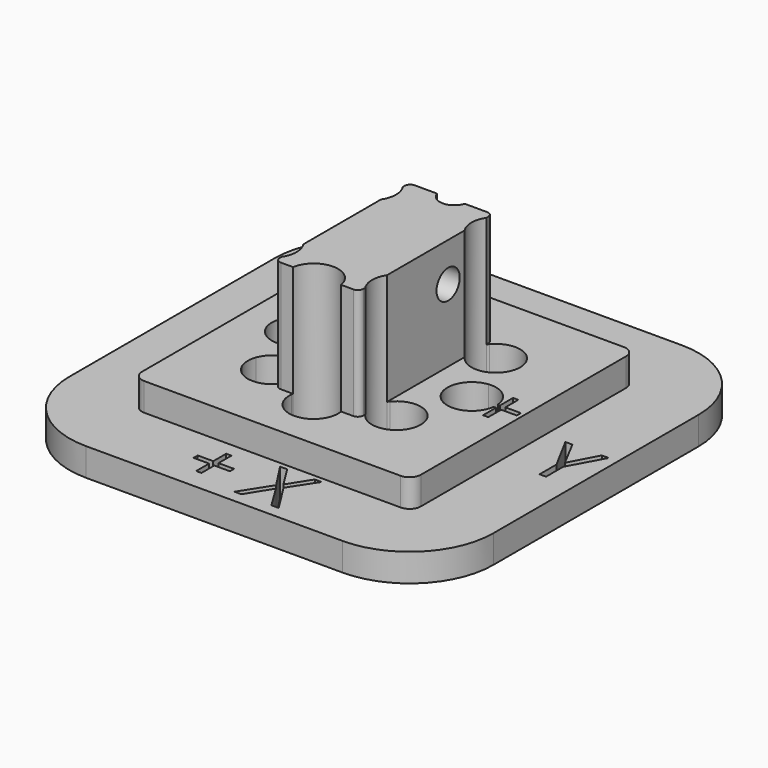
from build123d import *
from build123d import SkipClean  # not in build123d's __all__

# Parameters (mm, degrees)
F0_R      = 2.575
F1_DEPTH  = 10
F2_DEPTH  = 10
F4_START  = 5
F4_DEPTH  = 5
F7_DEPTH  = 30
F8_R      = 2.6
F9_DEPTH  = 12.5
F11_START = 5
F11_DEPTH = 5


# Not quite as in the source:
# - after a boolean that leaves OpenCascade's solid faulty, fix() repairs it


with BuildPart() as f1:
    # F0 (on Top) → F1 (new body)
    with BuildSketch(Plane.XY):
        with BuildLine():
            Line((23, 38), (-23, 38))
            ThreePointArc((-23, 38), (-33.6066017178, 33.6066017178), (-38, 23))
            Line((-38, 23), (-38, -23))
            ThreePointArc((-38, -23), (-33.6066017178, -33.6066017178), (-23, -38))
            Line((-23, -38), (23, -38))
            ThreePointArc((23, -38), (33.6066017178, -33.6066017178), (38, -23))
            Line((38, -23), (38, 23))
            ThreePointArc((38, 23), (33.6066017178, 33.6066017178), (23, 38))
        make_face()
        Polygon((-5.3266059028, -27.5300209804), (-5.3266059028, -30.4314966748), (-2.5336371528, -30.4314966748), (-2.5336371528, -31.3668265359), (-5.3266059028, -31.3668265359), (-5.3266059028, -34.2574515359), (-6.2706163194, -34.2574515359), (-6.2706163194, -31.3668265359), (-9.0505642361, -31.3668265359), (-9.0505642361, -30.4314966748), (-6.2706163194, -30.4314966748), (-6.2706163194, -27.5300209804), align=None, mode=Mode.SUBTRACT)
        Polygon((6.4463975694, -30.5747258415), (9.755859375, -35.7960800081), (8.447265625, -35.7960800081), (5.7823350694, -31.4362709804), (3.0696614583, -35.7960800081), (1.8478732639, -35.7960800081), (5.1443142361, -30.6137883415), (2.0713975694, -25.8807154248), (3.3474392361, -25.8807154248), (5.8083767361, -29.8086668137), (8.291015625, -25.8807154248), (9.5171440972, -25.8807154248), align=None, mode=Mode.SUBTRACT)
        Polygon((29.8459162505, 4.9153645833), (32.4717843061, -0.0434027778), (35.1150134727, 4.9153645833), (36.3628433338, 4.9153645833), (33.0533815283, -1.1545138889), (33.0533815283, -5), (31.888016945, -5), (31.888016945, -1.2087673611), (28.5850655561, 4.9153645833), align=None, mode=Mode.SUBTRACT)
        with BuildLine():
            ThreePointArc((-25, 23), (-24.4142135624, 24.4142135624), (-23, 25))
            Line((-23, 25), (23, 25))
            ThreePointArc((23, 25), (24.4142135624, 24.4142135624), (25, 23))
            Line((25, 23), (25, -23))
            ThreePointArc((25, -23), (24.4142135624, -24.4142135624), (23, -25))
            Line((23, -25), (-23, -25))
            ThreePointArc((-23, -25), (-24.4142135624, -24.4142135624), (-25, -23))
            Line((-25, -23), (-25, 23))
        make_face(mode=Mode.SUBTRACT)
        with BuildLine():
            Line((23, 25), (-23, 25))
            ThreePointArc((-23, 25), (-24.4142135624, 24.4142135624), (-25, 23))
            Line((-25, 23), (-25, -23))
            ThreePointArc((-25, -23), (-24.4142135624, -24.4142135624), (-23, -25))
            Line((-23, -25), (23, -25))
            ThreePointArc((23, -25), (24.4142135624, -24.4142135624), (25, -23))
            Line((25, -23), (25, 23))
            ThreePointArc((25, 23), (24.4142135624, 24.4142135624), (23, 25))
        make_face()
        with BuildLine():
            ThreePointArc((-15.25, 9.6458600373), (-15.5119318037, 11.1369318037), (-15.25, 12.6280035701))
            Line((-15.25, 12.6280035701), (-15.25, 14))
            ThreePointArc((-15.25, 14), (-12.6871843354, 20.1871843354), (-6.5, 22.75))
            Line((-6.5, 22.75), (6.5, 22.75))
            ThreePointArc((6.5, 22.75), (12.6871843354, 20.1871843354), (15.25, 14))
            Line((15.25, 14), (15.25, 12.6280035701))
            ThreePointArc((15.25, 12.6280035701), (15.4459513185, 11.893883467), (15.5119318037, 11.1369318037))
            ThreePointArc((15.5119318037, 11.1369318037), (15.4459513185, 10.3799801404), (15.25, 9.6458600373))
            Line((15.25, 9.6458600373), (15.25, 4.3463346627))
            ThreePointArc((15.25, 4.3463346627), (18.5227362424, 3.384162929), (20.1097825626, 0.3645833333))
            Line((20.1097825626, 0.3645833333), (20.520829445, 0.3645833333))
            Line((20.520829445, 0.3645833333), (20.520829445, 3.2660590278))
            Line((20.520829445, 3.2660590278), (21.4648398616, 3.2660590278))
            Line((21.4648398616, 3.2660590278), (21.4648398616, 0.3645833333))
            Line((21.4648398616, 0.3645833333), (24.2578086116, 0.3645833333))
            Line((24.2578086116, 0.3645833333), (24.2578086116, -0.5707465278))
            Line((24.2578086116, -0.5707465278), (21.4648398616, -0.5707465278))
            Line((21.4648398616, -0.5707465278), (21.4648398616, -3.4613715278))
            Line((21.4648398616, -3.4613715278), (20.520829445, -3.4613715278))
            Line((20.520829445, -3.4613715278), (20.520829445, -0.5707465278))
            Line((20.520829445, -0.5707465278), (20.0876114857, -0.5707465278))
            ThreePointArc((20.0876114857, -0.5707465278), (18.4417618617, -3.4489191176), (15.25, -4.3463346627))
            Line((15.25, -4.3463346627), (15.25, -9.6458600373))
            ThreePointArc((15.25, -9.6458600373), (15.4459513185, -10.3799801404), (15.5119318037, -11.1369318037))
            ThreePointArc((15.5119318037, -11.1369318037), (15.4459513185, -11.893883467), (15.25, -12.6280035701))
            Line((15.25, -12.6280035701), (15.25, -14))
            ThreePointArc((15.25, -14), (12.6871843354, -20.1871843354), (6.5, -22.75))
            Line((6.5, -22.75), (-6.5, -22.75))
            ThreePointArc((-6.5, -22.75), (-12.6871843354, -20.1871843354), (-15.25, -14))
            Line((-15.25, -14), (-15.25, -12.6280035701))
            ThreePointArc((-15.25, -12.6280035701), (-15.5119318037, -11.1369318037), (-15.25, -9.6458600373))
            Line((-15.25, -9.6458600373), (-15.25, -4.3463346627))
            ThreePointArc((-15.25, -4.3463346627), (-20.125, 0), (-15.25, 4.3463346627))
            Line((-15.25, 4.3463346627), (-15.25, 9.6458600373))
        make_face(mode=Mode.SUBTRACT)
        with BuildLine():
            Line((-4.3102349124, 15), (-6.5, 15))
            ThreePointArc((-6.5, 15), (-7.2071067812, 14.7071067812), (-7.5, 14))
            Line((-7.5, 14), (-7.5, 13.5686702878))
            ThreePointArc((-7.5, 13.5686702878), (-6.9505131886, 12.4075710835), (-6.7619318037, 11.1369318037))
            ThreePointArc((-6.7619318037, 11.1369318037), (-6.9505131886, 9.8662925239), (-7.5, 8.7051933195))
            Line((-7.5, 8.7051933195), (-7.5, -8.7051933195))
            ThreePointArc((-7.5, -8.7051933195), (-6.9505131886, -9.8662925239), (-6.7619318037, -11.1369318037))
            ThreePointArc((-6.7619318037, -11.1369318037), (-6.9505131886, -12.4075710835), (-7.5, -13.5686702878))
            Line((-7.5, -13.5686702878), (-7.5, -14))
            ThreePointArc((-7.5, -14), (-7.2071067812, -14.7071067812), (-6.5, -15))
            Line((-6.5, -15), (-4.3102349124, -15))
            ThreePointArc((-4.3102349124, -15), (0, -11.375), (4.3102349124, -15))
            Line((4.3102349124, -15), (6.5, -15))
            ThreePointArc((6.5, -15), (7.2071067812, -14.7071067812), (7.5, -14))
            Line((7.5, -14), (7.5, -13.5686702878))
            ThreePointArc((7.5, -13.5686702878), (6.7619318037, -11.1369318037), (7.5, -8.7051933195))
            Line((7.5, -8.7051933195), (7.5, 8.7051933195))
            ThreePointArc((7.5, 8.7051933195), (6.7619318037, 11.1369318037), (7.5, 13.5686702878))
            Line((7.5, 13.5686702878), (7.5, 14))
            ThreePointArc((7.5, 14), (7.2071067812, 14.7071067812), (6.5, 15))
            Line((6.5, 15), (4.3102349124, 15))
            ThreePointArc((4.3102349124, 15), (0, 11.375), (-4.3102349124, 15))
        make_face()
        with BuildLine():
            Line((-6.5, 15.25), (-4.3463346627, 15.25))
            ThreePointArc((-4.3463346627, 15.25), (-0.2504105137, 20.1178277867), (4.375, 15.75))
            ThreePointArc((4.375, 15.75), (4.3678277867, 15.4995894863), (4.3463346627, 15.25))
            Line((4.3463346627, 15.25), (6.5, 15.25))
            ThreePointArc((6.5, 15.25), (7.3838834765, 14.8838834765), (7.75, 14))
            Line((7.75, 14), (7.75, 13.9062851501))
            ThreePointArc((7.75, 13.9062851501), (11.8719960625, 15.4497389563), (15.25, 12.6280035701))
            Line((15.25, 12.6280035701), (15.25, 14))
            ThreePointArc((15.25, 14), (12.6871843354, 20.1871843354), (6.5, 22.75))
            Line((6.5, 22.75), (-6.5, 22.75))
            ThreePointArc((-6.5, 22.75), (-12.6871843354, 20.1871843354), (-15.25, 14))
            Line((-15.25, 14), (-15.25, 12.6280035701))
            ThreePointArc((-15.25, 12.6280035701), (-11.8719960625, 15.4497389563), (-7.75, 13.9062851501))
            Line((-7.75, 13.9062851501), (-7.75, 14))
            ThreePointArc((-7.75, 14), (-7.3838834765, 14.8838834765), (-6.5, 15.25))
        make_face()
        with BuildLine():
            Line((-7.75, -14), (-7.75, -13.9062851501))
            ThreePointArc((-7.75, -13.9062851501), (-11.8719960625, -15.4497389563), (-15.25, -12.6280035701))
            Line((-15.25, -12.6280035701), (-15.25, -14))
            ThreePointArc((-15.25, -14), (-12.6871843354, -20.1871843354), (-6.5, -22.75))
            Line((-6.5, -22.75), (6.5, -22.75))
            ThreePointArc((6.5, -22.75), (12.6871843354, -20.1871843354), (15.25, -14))
            Line((15.25, -14), (15.25, -12.6280035701))
            ThreePointArc((15.25, -12.6280035701), (11.8719960625, -15.4497389563), (7.75, -13.9062851501))
            Line((7.75, -13.9062851501), (7.75, -14))
            ThreePointArc((7.75, -14), (7.3838834765, -14.8838834765), (6.5, -15.25))
            Line((6.5, -15.25), (4.3463346627, -15.25))
            ThreePointArc((4.3463346627, -15.25), (4.3678277867, -15.4995894863), (4.375, -15.75))
            ThreePointArc((4.375, -15.75), (-0.2504105137, -20.1178277867), (-4.3463346627, -15.25))
            Line((-4.3463346627, -15.25), (-6.5, -15.25))
            ThreePointArc((-6.5, -15.25), (-7.3838834765, -14.8838834765), (-7.75, -14))
        make_face()
        with BuildLine():
            ThreePointArc((15.25, 9.6458600373), (11.8719960625, 6.8241246511), (7.75, 8.3675784573))
            Line((7.75, 8.3675784573), (7.75, -8.3675784573))
            ThreePointArc((7.75, -8.3675784573), (11.8719960625, -6.8241246511), (15.25, -9.6458600373))
            Line((15.25, -9.6458600373), (15.25, -4.3463346627))
            ThreePointArc((15.25, -4.3463346627), (11.375, 0), (15.25, 4.3463346627))
            Line((15.25, 4.3463346627), (15.25, 9.6458600373))
        make_face()
        with BuildLine():
            Line((-7.75, -8.3675784573), (-7.75, 8.3675784573))
            ThreePointArc((-7.75, 8.3675784573), (-11.8719960625, 6.8241246511), (-15.25, 9.6458600373))
            Line((-15.25, 9.6458600373), (-15.25, 4.3463346627))
            ThreePointArc((-15.25, 4.3463346627), (-12.4844123806, 2.9114536747), (-11.375, 0))
            ThreePointArc((-11.375, 0), (-12.4844123806, -2.9114536747), (-15.25, -4.3463346627))
            Line((-15.25, -4.3463346627), (-15.25, -9.6458600373))
            ThreePointArc((-15.25, -9.6458600373), (-11.8719960625, -6.8241246511), (-7.75, -8.3675784573))
        make_face()
        with BuildLine():
            ThreePointArc((15.25, 12.6280035701), (11.8719960625, 15.4497389563), (7.75, 13.9062851501))
            Line((7.75, 13.9062851501), (7.75, 8.3675784573))
            ThreePointArc((7.75, 8.3675784573), (11.8719960625, 6.8241246511), (15.25, 9.6458600373))
            Line((15.25, 9.6458600373), (15.25, 12.6280035701))
        make_face()
        with Locations((11.1369318037, 11.1369318037)):
            Circle(F0_R, mode=Mode.SUBTRACT)
        with BuildLine():
            Line((-7.75, 8.3675784573), (-7.75, 13.9062851501))
            ThreePointArc((-7.75, 13.9062851501), (-11.8719960625, 15.4497389563), (-15.25, 12.6280035701))
            Line((-15.25, 12.6280035701), (-15.25, 9.6458600373))
            ThreePointArc((-15.25, 9.6458600373), (-11.8719960625, 6.8241246511), (-7.75, 8.3675784573))
        make_face()
        with Locations((-11.1369318037, 11.1369318037)):
            Circle(F0_R, mode=Mode.SUBTRACT)
        with BuildLine():
            Line((-7.75, -13.9062851501), (-7.75, -8.3675784573))
            ThreePointArc((-7.75, -8.3675784573), (-11.8719960625, -6.8241246511), (-15.25, -9.6458600373))
            Line((-15.25, -9.6458600373), (-15.25, -12.6280035701))
            ThreePointArc((-15.25, -12.6280035701), (-11.8719960625, -15.4497389563), (-7.75, -13.9062851501))
        make_face()
        with Locations((-11.1369318037, -11.1369318037)):
            Circle(F0_R, mode=Mode.SUBTRACT)
        with BuildLine():
            ThreePointArc((15.25, -9.6458600373), (11.8719960625, -6.8241246511), (7.75, -8.3675784573))
            Line((7.75, -8.3675784573), (7.75, -13.9062851501))
            ThreePointArc((7.75, -13.9062851501), (11.8719960625, -15.4497389563), (15.25, -12.6280035701))
            Line((15.25, -12.6280035701), (15.25, -9.6458600373))
        make_face()
        with Locations((11.1369318037, -11.1369318037)):
            Circle(F0_R, mode=Mode.SUBTRACT)
        with BuildLine():
            ThreePointArc((4.375, 15.75), (-0.2504105137, 20.1178277867), (-4.3463346627, 15.25))
            Line((-4.3463346627, 15.25), (-2.525989905, 15.25))
            ThreePointArc((-2.525989905, 15.25), (-0.2511981237, 18.3127181863), (2.575, 15.75))
            ThreePointArc((2.575, 15.75), (2.5627181863, 15.4988018763), (2.525989905, 15.25))
            Line((2.525989905, 15.25), (4.3463346627, 15.25))
            ThreePointArc((4.3463346627, 15.25), (4.3678277867, 15.4995894863), (4.375, 15.75))
        make_face()
        with BuildLine():
            Line((-15.25, 2.525989905), (-15.25, 4.3463346627))
            ThreePointArc((-15.25, 4.3463346627), (-20.125, 0), (-15.25, -4.3463346627))
            Line((-15.25, -4.3463346627), (-15.25, -2.525989905))
            ThreePointArc((-15.25, -2.525989905), (-18.325, 0), (-15.25, 2.525989905))
        make_face()
        with BuildLine():
            Line((-2.525989905, -15.25), (-4.3463346627, -15.25))
            ThreePointArc((-4.3463346627, -15.25), (-0.2504105137, -20.1178277867), (4.375, -15.75))
            ThreePointArc((4.375, -15.75), (4.3678277867, -15.4995894863), (4.3463346627, -15.25))
            Line((4.3463346627, -15.25), (2.525989905, -15.25))
            ThreePointArc((2.525989905, -15.25), (2.5627181863, -15.4988018763), (2.575, -15.75))
            ThreePointArc((2.575, -15.75), (-0.2511981237, -18.3127181863), (-2.525989905, -15.25))
        make_face()
        with Locations((11.1369318037, 11.1369318037)):
            Circle(F0_R)
        with Locations((-11.1369318037, 11.1369318037)):
            Circle(F0_R)
        with Locations((-11.1369318037, -11.1369318037)):
            Circle(F0_R)
        with Locations((11.1369318037, -11.1369318037)):
            Circle(F0_R)
        with BuildLine():
            ThreePointArc((-11.375, 0), (-12.4844123806, 2.9114536747), (-15.25, 4.3463346627))
            Line((-15.25, 4.3463346627), (-15.25, 2.525989905))
            ThreePointArc((-15.25, 2.525989905), (-13.7602606955, 1.6344915111), (-13.175, 0))
            ThreePointArc((-13.175, 0), (-13.7602606955, -1.6344915111), (-15.25, -2.525989905))
            Line((-15.25, -2.525989905), (-15.25, -4.3463346627))
            ThreePointArc((-15.25, -4.3463346627), (-12.4844123806, -2.9114536747), (-11.375, 0))
        make_face()
        with BuildLine():
            Line((15.25, 2.525989905), (15.25, 4.3463346627))
            ThreePointArc((15.25, 4.3463346627), (11.375, 0), (15.25, -4.3463346627))
            Line((15.25, -4.3463346627), (15.25, -2.525989905))
            ThreePointArc((15.25, -2.525989905), (13.175, 0), (15.25, 2.525989905))
        make_face()
        with BuildLine():
            Line((-2.46335645, 15), (-4.3102349124, 15))
            ThreePointArc((-4.3102349124, 15), (0, 11.375), (4.3102349124, 15))
            Line((4.3102349124, 15), (2.46335645, 15))
            ThreePointArc((2.46335645, 15), (0, 13.175), (-2.46335645, 15))
        make_face()
        with BuildLine():
            ThreePointArc((4.3102349124, -15), (0, -11.375), (-4.3102349124, -15))
            Line((-4.3102349124, -15), (-2.46335645, -15))
            ThreePointArc((-2.46335645, -15), (0, -13.175), (2.46335645, -15))
            Line((2.46335645, -15), (4.3102349124, -15))
        make_face()
        with BuildLine():
            ThreePointArc((2.575, 15.75), (-0.2511981237, 18.3127181863), (-2.525989905, 15.25))
            Line((-2.525989905, 15.25), (2.525989905, 15.25))
            ThreePointArc((2.525989905, 15.25), (2.5627181863, 15.4988018763), (2.575, 15.75))
        make_face()
        with BuildLine():
            Line((-15.25, -2.525989905), (-15.25, 2.525989905))
            ThreePointArc((-15.25, 2.525989905), (-18.325, 0), (-15.25, -2.525989905))
        make_face()
        with BuildLine():
            Line((2.525989905, -15.25), (-2.525989905, -15.25))
            ThreePointArc((-2.525989905, -15.25), (-0.2511981237, -18.3127181863), (2.575, -15.75))
            ThreePointArc((2.575, -15.75), (2.5627181863, -15.4988018763), (2.525989905, -15.25))
        make_face()
        with BuildLine():
            ThreePointArc((18.299059433, 0.3645833333), (17.2391543681, 2.1007247007), (15.25, 2.525989905))
            Line((15.25, 2.525989905), (15.25, -2.525989905))
            ThreePointArc((15.25, -2.525989905), (17.1523996727, -2.1596064822), (18.2609506967, -0.5707465278))
            Line((18.2609506967, -0.5707465278), (17.7408815283, -0.5707465278))
            Line((17.7408815283, -0.5707465278), (17.7408815283, 0.3645833333))
            Line((17.7408815283, 0.3645833333), (18.299059433, 0.3645833333))
        make_face()
        with BuildLine():
            ThreePointArc((20.1097825626, 0.3645833333), (18.5227362424, 3.384162929), (15.25, 4.3463346627))
            Line((15.25, 4.3463346627), (15.25, 2.525989905))
            ThreePointArc((15.25, 2.525989905), (17.2391543681, 2.1007247007), (18.299059433, 0.3645833333))
            Line((18.299059433, 0.3645833333), (20.1097825626, 0.3645833333))
        make_face()
        with BuildLine():
            Line((15.25, -2.525989905), (15.25, -4.3463346627))
            ThreePointArc((15.25, -4.3463346627), (18.4417618617, -3.4489191176), (20.0876114857, -0.5707465278))
            Line((20.0876114857, -0.5707465278), (18.2609506967, -0.5707465278))
            ThreePointArc((18.2609506967, -0.5707465278), (17.1523996727, -2.1596064822), (15.25, -2.525989905))
        make_face()
        with BuildLine():
            ThreePointArc((-13.175, 0), (-13.7602606955, 1.6344915111), (-15.25, 2.525989905))
            Line((-15.25, 2.525989905), (-15.25, -2.525989905))
            ThreePointArc((-15.25, -2.525989905), (-13.7602606955, -1.6344915111), (-13.175, 0))
        make_face()
        with BuildLine():
            Line((15.25, -2.525989905), (15.25, 2.525989905))
            ThreePointArc((15.25, 2.525989905), (13.175, 0), (15.25, -2.525989905))
        make_face()
        with BuildLine():
            ThreePointArc((2.46335645, -15), (0, -13.175), (-2.46335645, -15))
            Line((-2.46335645, -15), (2.46335645, -15))
        make_face()
        with BuildLine():
            Line((2.46335645, 15), (-2.46335645, 15))
            ThreePointArc((-2.46335645, 15), (0, 13.175), (2.46335645, 15))
        make_face()
        with BuildLine():
            ThreePointArc((7.75, 8.3675784573), (7.6209453216, 8.5333834447), (7.5, 8.7051933195))
            Line((7.5, 8.7051933195), (7.5, -8.7051933195))
            ThreePointArc((7.5, -8.7051933195), (7.6209453216, -8.5333834447), (7.75, -8.3675784573))
            Line((7.75, -8.3675784573), (7.75, 8.3675784573))
        make_face()
        with BuildLine():
            Line((-7.5, -8.7051933195), (-7.5, 8.7051933195))
            ThreePointArc((-7.5, 8.7051933195), (-7.6209453216, 8.5333834447), (-7.75, 8.3675784573))
            Line((-7.75, 8.3675784573), (-7.75, -8.3675784573))
            ThreePointArc((-7.75, -8.3675784573), (-7.6209453216, -8.5333834447), (-7.5, -8.7051933195))
        make_face()
        with BuildLine():
            ThreePointArc((-6.7619318037, -11.1369318037), (-6.9505131886, -9.8662925239), (-7.5, -8.7051933195))
            Line((-7.5, -8.7051933195), (-7.5, -13.5686702878))
            ThreePointArc((-7.5, -13.5686702878), (-6.9505131886, -12.4075710835), (-6.7619318037, -11.1369318037))
        make_face()
        with BuildLine():
            Line((7.5, -13.5686702878), (7.5, -8.7051933195))
            ThreePointArc((7.5, -8.7051933195), (6.7619318037, -11.1369318037), (7.5, -13.5686702878))
        make_face()
        with BuildLine():
            Line((7.5, 8.7051933195), (7.5, 13.5686702878))
            ThreePointArc((7.5, 13.5686702878), (6.7619318037, 11.1369318037), (7.5, 8.7051933195))
        make_face()
        with BuildLine():
            ThreePointArc((-6.7619318037, 11.1369318037), (-6.9505131886, 12.4075710835), (-7.5, 13.5686702878))
            Line((-7.5, 13.5686702878), (-7.5, 8.7051933195))
            ThreePointArc((-7.5, 8.7051933195), (-6.9505131886, 9.8662925239), (-6.7619318037, 11.1369318037))
        make_face()
        with BuildLine():
            ThreePointArc((7.75, 13.9062851501), (7.6209453216, 13.7404801626), (7.5, 13.5686702878))
            Line((7.5, 13.5686702878), (7.5, 8.7051933195))
            ThreePointArc((7.5, 8.7051933195), (7.6209453216, 8.5333834447), (7.75, 8.3675784573))
            Line((7.75, 8.3675784573), (7.75, 13.9062851501))
        make_face()
        with BuildLine():
            ThreePointArc((7.75, -8.3675784573), (7.6209453216, -8.5333834447), (7.5, -8.7051933195))
            Line((7.5, -8.7051933195), (7.5, -13.5686702878))
            ThreePointArc((7.5, -13.5686702878), (7.6209453216, -13.7404801626), (7.75, -13.9062851501))
            Line((7.75, -13.9062851501), (7.75, -8.3675784573))
        make_face()
        with BuildLine():
            Line((-7.5, 8.7051933195), (-7.5, 13.5686702878))
            ThreePointArc((-7.5, 13.5686702878), (-7.6209453216, 13.7404801626), (-7.75, 13.9062851501))
            Line((-7.75, 13.9062851501), (-7.75, 8.3675784573))
            ThreePointArc((-7.75, 8.3675784573), (-7.6209453216, 8.5333834447), (-7.5, 8.7051933195))
        make_face()
        with BuildLine():
            Line((-7.5, -13.5686702878), (-7.5, -8.7051933195))
            ThreePointArc((-7.5, -8.7051933195), (-7.6209453216, -8.5333834447), (-7.75, -8.3675784573))
            Line((-7.75, -8.3675784573), (-7.75, -13.9062851501))
            ThreePointArc((-7.75, -13.9062851501), (-7.6209453216, -13.7404801626), (-7.5, -13.5686702878))
        make_face()
        with BuildLine():
            ThreePointArc((-2.525989905, 15.25), (-2.4978028871, 15.1242159019), (-2.46335645, 15))
            Line((-2.46335645, 15), (2.46335645, 15))
            ThreePointArc((2.46335645, 15), (2.4978028871, 15.1242159019), (2.525989905, 15.25))
            Line((2.525989905, 15.25), (-2.525989905, 15.25))
        make_face()
        with BuildLine():
            Line((2.46335645, -15), (-2.46335645, -15))
            ThreePointArc((-2.46335645, -15), (-2.4978028871, -15.1242159019), (-2.525989905, -15.25))
            Line((-2.525989905, -15.25), (2.525989905, -15.25))
            ThreePointArc((2.525989905, -15.25), (2.4978028871, -15.1242159019), (2.46335645, -15))
        make_face()
        with BuildLine():
            ThreePointArc((4.3463346627, 15.25), (4.3300893988, 15.1247394159), (4.3102349124, 15))
            Line((4.3102349124, 15), (6.5, 15))
            ThreePointArc((6.5, 15), (7.2071067812, 14.7071067812), (7.5, 14))
            Line((7.5, 14), (7.5, 13.5686702878))
            ThreePointArc((7.5, 13.5686702878), (7.6209453216, 13.7404801626), (7.75, 13.9062851501))
            Line((7.75, 13.9062851501), (7.75, 14))
            ThreePointArc((7.75, 14), (7.3838834765, 14.8838834765), (6.5, 15.25))
            Line((6.5, 15.25), (4.3463346627, 15.25))
        make_face()
        with BuildLine():
            ThreePointArc((7.75, -13.9062851501), (7.6209453216, -13.7404801626), (7.5, -13.5686702878))
            Line((7.5, -13.5686702878), (7.5, -14))
            ThreePointArc((7.5, -14), (7.2071067812, -14.7071067812), (6.5, -15))
            Line((6.5, -15), (4.3102349124, -15))
            ThreePointArc((4.3102349124, -15), (4.3300893988, -15.1247394159), (4.3463346627, -15.25))
            Line((4.3463346627, -15.25), (6.5, -15.25))
            ThreePointArc((6.5, -15.25), (7.3838834765, -14.8838834765), (7.75, -14))
            Line((7.75, -14), (7.75, -13.9062851501))
        make_face()
        with BuildLine():
            ThreePointArc((-7.5, 14), (-7.2071067812, 14.7071067812), (-6.5, 15))
            Line((-6.5, 15), (-4.3102349124, 15))
            ThreePointArc((-4.3102349124, 15), (-4.3300893988, 15.1247394159), (-4.3463346627, 15.25))
            Line((-4.3463346627, 15.25), (-6.5, 15.25))
            ThreePointArc((-6.5, 15.25), (-7.3838834765, 14.8838834765), (-7.75, 14))
            Line((-7.75, 14), (-7.75, 13.9062851501))
            ThreePointArc((-7.75, 13.9062851501), (-7.6209453216, 13.7404801626), (-7.5, 13.5686702878))
            Line((-7.5, 13.5686702878), (-7.5, 14))
        make_face()
        with BuildLine():
            Line((-7.5, -14), (-7.5, -13.5686702878))
            ThreePointArc((-7.5, -13.5686702878), (-7.6209453216, -13.7404801626), (-7.75, -13.9062851501))
            Line((-7.75, -13.9062851501), (-7.75, -14))
            ThreePointArc((-7.75, -14), (-7.3838834765, -14.8838834765), (-6.5, -15.25))
            Line((-6.5, -15.25), (-4.3463346627, -15.25))
            ThreePointArc((-4.3463346627, -15.25), (-4.3300893988, -15.1247394159), (-4.3102349124, -15))
            Line((-4.3102349124, -15), (-6.5, -15))
            ThreePointArc((-6.5, -15), (-7.2071067812, -14.7071067812), (-7.5, -14))
        make_face()
        with BuildLine():
            Line((-15.25, 9.6458600373), (-15.25, 12.6280035701))
            ThreePointArc((-15.25, 12.6280035701), (-15.5119318037, 11.1369318037), (-15.25, 9.6458600373))
        make_face()
        with BuildLine():
            ThreePointArc((15.5119318037, 11.1369318037), (15.4459513185, 11.893883467), (15.25, 12.6280035701))
            Line((15.25, 12.6280035701), (15.25, 9.6458600373))
            ThreePointArc((15.25, 9.6458600373), (15.4459513185, 10.3799801404), (15.5119318037, 11.1369318037))
        make_face()
        with BuildLine():
            Line((-15.25, -12.6280035701), (-15.25, -9.6458600373))
            ThreePointArc((-15.25, -9.6458600373), (-15.5119318037, -11.1369318037), (-15.25, -12.6280035701))
        make_face()
        with BuildLine():
            ThreePointArc((15.5119318037, -11.1369318037), (15.4459513185, -10.3799801404), (15.25, -9.6458600373))
            Line((15.25, -9.6458600373), (15.25, -12.6280035701))
            ThreePointArc((15.25, -12.6280035701), (15.4459513185, -11.893883467), (15.5119318037, -11.1369318037))
        make_face()
        with BuildLine():
            ThreePointArc((-4.3463346627, 15.25), (-4.3300893988, 15.1247394159), (-4.3102349124, 15))
            Line((-4.3102349124, 15), (-2.46335645, 15))
            ThreePointArc((-2.46335645, 15), (-2.4978028871, 15.1242159019), (-2.525989905, 15.25))
            Line((-2.525989905, 15.25), (-4.3463346627, 15.25))
        make_face()
        with BuildLine():
            Line((2.46335645, 15), (4.3102349124, 15))
            ThreePointArc((4.3102349124, 15), (4.3300893988, 15.1247394159), (4.3463346627, 15.25))
            Line((4.3463346627, 15.25), (2.525989905, 15.25))
            ThreePointArc((2.525989905, 15.25), (2.4978028871, 15.1242159019), (2.46335645, 15))
        make_face()
        with BuildLine():
            Line((-2.46335645, -15), (-4.3102349124, -15))
            ThreePointArc((-4.3102349124, -15), (-4.3300893988, -15.1247394159), (-4.3463346627, -15.25))
            Line((-4.3463346627, -15.25), (-2.525989905, -15.25))
            ThreePointArc((-2.525989905, -15.25), (-2.4978028871, -15.1242159019), (-2.46335645, -15))
        make_face()
        with BuildLine():
            ThreePointArc((4.3463346627, -15.25), (4.3300893988, -15.1247394159), (4.3102349124, -15))
            Line((4.3102349124, -15), (2.46335645, -15))
            ThreePointArc((2.46335645, -15), (2.4978028871, -15.1242159019), (2.525989905, -15.25))
            Line((2.525989905, -15.25), (4.3463346627, -15.25))
        make_face()
    extrude(amount=F1_DEPTH)


with BuildPart() as f2:
    # F0 (on Top) → F2 (new body)
    with BuildSketch(Plane.XY):
        with BuildLine():
            Line((2.46335645, 15), (-2.46335645, 15))
            ThreePointArc((-2.46335645, 15), (0, 13.175), (2.46335645, 15))
        make_face()
        with BuildLine():
            ThreePointArc((2.575, 15.75), (-0.2511981237, 18.3127181863), (-2.525989905, 15.25))
            Line((-2.525989905, 15.25), (2.525989905, 15.25))
            ThreePointArc((2.525989905, 15.25), (2.5627181863, 15.4988018763), (2.575, 15.75))
        make_face()
        with BuildLine():
            ThreePointArc((-2.525989905, 15.25), (-2.4978028871, 15.1242159019), (-2.46335645, 15))
            Line((-2.46335645, 15), (2.46335645, 15))
            ThreePointArc((2.46335645, 15), (2.4978028871, 15.1242159019), (2.525989905, 15.25))
            Line((2.525989905, 15.25), (-2.525989905, 15.25))
        make_face()
    extrude(amount=F2_DEPTH)


with BuildPart() as f2b:
    # F0 (on Top) → F2, piece 2 (new body)
    with BuildSketch(Plane.XY):
        with Locations((-11.1369318037, 11.1369318037)):
            Circle(F0_R)
    extrude(amount=F2_DEPTH)


with BuildPart() as f2c:
    # F0 (on Top) → F2, piece 3 (new body)
    with BuildSketch(Plane.XY):
        with BuildLine():
            Line((-15.25, -2.525989905), (-15.25, 2.525989905))
            ThreePointArc((-15.25, 2.525989905), (-18.325, 0), (-15.25, -2.525989905))
        make_face()
        with BuildLine():
            ThreePointArc((-13.175, 0), (-13.7602606955, 1.6344915111), (-15.25, 2.525989905))
            Line((-15.25, 2.525989905), (-15.25, -2.525989905))
            ThreePointArc((-15.25, -2.525989905), (-13.7602606955, -1.6344915111), (-13.175, 0))
        make_face()
    extrude(amount=F2_DEPTH)


with BuildPart() as f2d:
    # F0 (on Top) → F2, piece 4 (new body)
    with BuildSketch(Plane.XY):
        with Locations((11.1369318037, 11.1369318037)):
            Circle(F0_R)
    extrude(amount=F2_DEPTH)


with BuildPart() as f2e:
    # F0 (on Top) → F2, piece 5 (new body)
    with BuildSketch(Plane.XY):
        with BuildLine():
            ThreePointArc((18.299059433, 0.3645833333), (17.2391543681, 2.1007247007), (15.25, 2.525989905))
            Line((15.25, 2.525989905), (15.25, -2.525989905))
            ThreePointArc((15.25, -2.525989905), (17.1523996727, -2.1596064822), (18.2609506967, -0.5707465278))
            Line((18.2609506967, -0.5707465278), (17.7408815283, -0.5707465278))
            Line((17.7408815283, -0.5707465278), (17.7408815283, 0.3645833333))
            Line((17.7408815283, 0.3645833333), (18.299059433, 0.3645833333))
        make_face()
        with BuildLine():
            Line((15.25, -2.525989905), (15.25, 2.525989905))
            ThreePointArc((15.25, 2.525989905), (13.175, 0), (15.25, -2.525989905))
        make_face()
        with BuildLine():
            ThreePointArc((18.325, 0), (18.3185066712, 0.1827525102), (18.299059433, 0.3645833333))
            Line((18.299059433, 0.3645833333), (17.7408815283, 0.3645833333))
            Line((17.7408815283, 0.3645833333), (17.7408815283, -0.5707465278))
            Line((17.7408815283, -0.5707465278), (18.2609506967, -0.5707465278))
            ThreePointArc((18.2609506967, -0.5707465278), (18.3089375768, -0.2871645487), (18.325, 0))
        make_face()
    extrude(amount=F2_DEPTH)


with BuildPart() as f2f:
    # F0 (on Top) → F2, piece 6 (new body)
    with BuildSketch(Plane.XY):
        with Locations((11.1369318037, -11.1369318037)):
            Circle(F0_R)
    extrude(amount=F2_DEPTH)


with BuildPart() as f2g:
    # F0 (on Top) → F2, piece 7 (new body)
    with BuildSketch(Plane.XY):
        with Locations((-11.1369318037, -11.1369318037)):
            Circle(F0_R)
    extrude(amount=F2_DEPTH)


with BuildPart() as f2h:
    # F0 (on Top) → F2, piece 8 (new body)
    with BuildSketch(Plane.XY):
        with BuildLine():
            ThreePointArc((2.46335645, -15), (0, -13.175), (-2.46335645, -15))
            Line((-2.46335645, -15), (2.46335645, -15))
        make_face()
        with BuildLine():
            Line((2.525989905, -15.25), (-2.525989905, -15.25))
            ThreePointArc((-2.525989905, -15.25), (-0.2511981237, -18.3127181863), (2.575, -15.75))
            ThreePointArc((2.575, -15.75), (2.5627181863, -15.4988018763), (2.525989905, -15.25))
        make_face()
        with BuildLine():
            Line((2.46335645, -15), (-2.46335645, -15))
            ThreePointArc((-2.46335645, -15), (-2.4978028871, -15.1242159019), (-2.525989905, -15.25))
            Line((-2.525989905, -15.25), (2.525989905, -15.25))
            ThreePointArc((2.525989905, -15.25), (2.4978028871, -15.1242159019), (2.46335645, -15))
        make_face()
    extrude(amount=F2_DEPTH)


with BuildPart() as f1_1:
    add(f1.part, clean=False)

    # F3: cut F2, F2b, F2c, F2g, F2h, F2f, F2d, F2e
    add(f2.part, mode=Mode.SUBTRACT)
    add(f2b.part, mode=Mode.SUBTRACT)
    add(f2c.part, mode=Mode.SUBTRACT)
    add(f2g.part, mode=Mode.SUBTRACT)
    add(f2h.part, mode=Mode.SUBTRACT)
    add(f2f.part, mode=Mode.SUBTRACT)
    add(f2d.part, mode=Mode.SUBTRACT)
    add(f2e.part, mode=Mode.SUBTRACT)


with BuildPart() as f4:
    # F0 (on Top) → F4 (new body)
    with BuildSketch(Plane.XY.offset(F4_START)):
        with BuildLine():
            ThreePointArc((20.125, 0), (20.1211939851, 0.1824503887), (20.1097825626, 0.3645833333))
            Line((20.1097825626, 0.3645833333), (18.299059433, 0.3645833333))
            ThreePointArc((18.299059433, 0.3645833333), (18.3185066712, 0.1827525102), (18.325, 0))
            ThreePointArc((18.325, 0), (18.3089375768, -0.2871645487), (18.2609506967, -0.5707465278))
            Line((18.2609506967, -0.5707465278), (20.0876114857, -0.5707465278))
            ThreePointArc((20.0876114857, -0.5707465278), (20.115642865, -0.2859849209), (20.125, 0))
        make_face()
        with BuildLine():
            ThreePointArc((20.1097825626, 0.3645833333), (18.5227362424, 3.384162929), (15.25, 4.3463346627))
            Line((15.25, 4.3463346627), (15.25, 2.525989905))
            ThreePointArc((15.25, 2.525989905), (17.2391543681, 2.1007247007), (18.299059433, 0.3645833333))
            Line((18.299059433, 0.3645833333), (20.1097825626, 0.3645833333))
        make_face()
        with BuildLine():
            ThreePointArc((18.299059433, 0.3645833333), (17.2391543681, 2.1007247007), (15.25, 2.525989905))
            Line((15.25, 2.525989905), (15.25, -2.525989905))
            ThreePointArc((15.25, -2.525989905), (17.1523996727, -2.1596064822), (18.2609506967, -0.5707465278))
            Line((18.2609506967, -0.5707465278), (17.7408815283, -0.5707465278))
            Line((17.7408815283, -0.5707465278), (17.7408815283, 0.3645833333))
            Line((17.7408815283, 0.3645833333), (18.299059433, 0.3645833333))
        make_face()
        with BuildLine():
            ThreePointArc((18.325, 0), (18.3185066712, 0.1827525102), (18.299059433, 0.3645833333))
            Line((18.299059433, 0.3645833333), (17.7408815283, 0.3645833333))
            Line((17.7408815283, 0.3645833333), (17.7408815283, -0.5707465278))
            Line((17.7408815283, -0.5707465278), (18.2609506967, -0.5707465278))
            ThreePointArc((18.2609506967, -0.5707465278), (18.3089375768, -0.2871645487), (18.325, 0))
        make_face()
        with BuildLine():
            Line((15.25, -2.525989905), (15.25, -4.3463346627))
            ThreePointArc((15.25, -4.3463346627), (18.4417618617, -3.4489191176), (20.0876114857, -0.5707465278))
            Line((20.0876114857, -0.5707465278), (18.2609506967, -0.5707465278))
            ThreePointArc((18.2609506967, -0.5707465278), (17.1523996727, -2.1596064822), (15.25, -2.525989905))
        make_face()
        with BuildLine():
            Line((15.25, 2.525989905), (15.25, 4.3463346627))
            ThreePointArc((15.25, 4.3463346627), (11.375, 0), (15.25, -4.3463346627))
            Line((15.25, -4.3463346627), (15.25, -2.525989905))
            ThreePointArc((15.25, -2.525989905), (13.175, 0), (15.25, 2.525989905))
        make_face()
        with BuildLine():
            Line((15.25, -2.525989905), (15.25, 2.525989905))
            ThreePointArc((15.25, 2.525989905), (13.175, 0), (15.25, -2.525989905))
        make_face()
    extrude(amount=F4_DEPTH)


with BuildPart() as f4b:
    # F0 (on Top) → F4, piece 2 (new body)
    with BuildSketch(Plane.XY.offset(F4_START)):
        with BuildLine():
            ThreePointArc((15.25, 12.6280035701), (11.8719960625, 15.4497389563), (7.75, 13.9062851501))
            Line((7.75, 13.9062851501), (7.75, 8.3675784573))
            ThreePointArc((7.75, 8.3675784573), (11.8719960625, 6.8241246511), (15.25, 9.6458600373))
            Line((15.25, 9.6458600373), (15.25, 12.6280035701))
        make_face()
        with Locations((11.1369318037, 11.1369318037)):
            Circle(F0_R, mode=Mode.SUBTRACT)
        with BuildLine():
            ThreePointArc((15.5119318037, 11.1369318037), (15.4459513185, 11.893883467), (15.25, 12.6280035701))
            Line((15.25, 12.6280035701), (15.25, 9.6458600373))
            ThreePointArc((15.25, 9.6458600373), (15.4459513185, 10.3799801404), (15.5119318037, 11.1369318037))
        make_face()
        with BuildLine():
            Line((7.5, 8.7051933195), (7.5, 13.5686702878))
            ThreePointArc((7.5, 13.5686702878), (6.7619318037, 11.1369318037), (7.5, 8.7051933195))
        make_face()
        with BuildLine():
            ThreePointArc((7.75, 13.9062851501), (7.6209453216, 13.7404801626), (7.5, 13.5686702878))
            Line((7.5, 13.5686702878), (7.5, 8.7051933195))
            ThreePointArc((7.5, 8.7051933195), (7.6209453216, 8.5333834447), (7.75, 8.3675784573))
            Line((7.75, 8.3675784573), (7.75, 13.9062851501))
        make_face()
        with Locations((11.1369318037, 11.1369318037)):
            Circle(F0_R)
    extrude(amount=F4_DEPTH)


with BuildPart() as f4c:
    # F0 (on Top) → F4, piece 3 (new body)
    with BuildSketch(Plane.XY.offset(F4_START)):
        with BuildLine():
            Line((-2.46335645, 15), (-4.3102349124, 15))
            ThreePointArc((-4.3102349124, 15), (0, 11.375), (4.3102349124, 15))
            Line((4.3102349124, 15), (2.46335645, 15))
            ThreePointArc((2.46335645, 15), (0, 13.175), (-2.46335645, 15))
        make_face()
        with BuildLine():
            Line((2.46335645, 15), (-2.46335645, 15))
            ThreePointArc((-2.46335645, 15), (0, 13.175), (2.46335645, 15))
        make_face()
        with BuildLine():
            ThreePointArc((2.575, 15.75), (-0.2511981237, 18.3127181863), (-2.525989905, 15.25))
            Line((-2.525989905, 15.25), (2.525989905, 15.25))
            ThreePointArc((2.525989905, 15.25), (2.5627181863, 15.4988018763), (2.575, 15.75))
        make_face()
        with BuildLine():
            ThreePointArc((4.375, 15.75), (-0.2504105137, 20.1178277867), (-4.3463346627, 15.25))
            Line((-4.3463346627, 15.25), (-2.525989905, 15.25))
            ThreePointArc((-2.525989905, 15.25), (-0.2511981237, 18.3127181863), (2.575, 15.75))
            ThreePointArc((2.575, 15.75), (2.5627181863, 15.4988018763), (2.525989905, 15.25))
            Line((2.525989905, 15.25), (4.3463346627, 15.25))
            ThreePointArc((4.3463346627, 15.25), (4.3678277867, 15.4995894863), (4.375, 15.75))
        make_face()
        with BuildLine():
            Line((2.46335645, 15), (4.3102349124, 15))
            ThreePointArc((4.3102349124, 15), (4.3300893988, 15.1247394159), (4.3463346627, 15.25))
            Line((4.3463346627, 15.25), (2.525989905, 15.25))
            ThreePointArc((2.525989905, 15.25), (2.4978028871, 15.1242159019), (2.46335645, 15))
        make_face()
        with BuildLine():
            ThreePointArc((-2.525989905, 15.25), (-2.4978028871, 15.1242159019), (-2.46335645, 15))
            Line((-2.46335645, 15), (2.46335645, 15))
            ThreePointArc((2.46335645, 15), (2.4978028871, 15.1242159019), (2.525989905, 15.25))
            Line((2.525989905, 15.25), (-2.525989905, 15.25))
        make_face()
        with BuildLine():
            ThreePointArc((-4.3463346627, 15.25), (-4.3300893988, 15.1247394159), (-4.3102349124, 15))
            Line((-4.3102349124, 15), (-2.46335645, 15))
            ThreePointArc((-2.46335645, 15), (-2.4978028871, 15.1242159019), (-2.525989905, 15.25))
            Line((-2.525989905, 15.25), (-4.3463346627, 15.25))
        make_face()
    extrude(amount=F4_DEPTH)


with BuildPart() as f4d:
    # F0 (on Top) → F4, piece 4 (new body)
    with BuildSketch(Plane.XY.offset(F4_START)):
        with BuildLine():
            Line((-7.75, 8.3675784573), (-7.75, 13.9062851501))
            ThreePointArc((-7.75, 13.9062851501), (-11.8719960625, 15.4497389563), (-15.25, 12.6280035701))
            Line((-15.25, 12.6280035701), (-15.25, 9.6458600373))
            ThreePointArc((-15.25, 9.6458600373), (-11.8719960625, 6.8241246511), (-7.75, 8.3675784573))
        make_face()
        with Locations((-11.1369318037, 11.1369318037)):
            Circle(F0_R, mode=Mode.SUBTRACT)
        with Locations((-11.1369318037, 11.1369318037)):
            Circle(F0_R)
        with BuildLine():
            Line((-7.5, 8.7051933195), (-7.5, 13.5686702878))
            ThreePointArc((-7.5, 13.5686702878), (-7.6209453216, 13.7404801626), (-7.75, 13.9062851501))
            Line((-7.75, 13.9062851501), (-7.75, 8.3675784573))
            ThreePointArc((-7.75, 8.3675784573), (-7.6209453216, 8.5333834447), (-7.5, 8.7051933195))
        make_face()
        with BuildLine():
            ThreePointArc((-6.7619318037, 11.1369318037), (-6.9505131886, 12.4075710835), (-7.5, 13.5686702878))
            Line((-7.5, 13.5686702878), (-7.5, 8.7051933195))
            ThreePointArc((-7.5, 8.7051933195), (-6.9505131886, 9.8662925239), (-6.7619318037, 11.1369318037))
        make_face()
        with BuildLine():
            Line((-15.25, 9.6458600373), (-15.25, 12.6280035701))
            ThreePointArc((-15.25, 12.6280035701), (-15.5119318037, 11.1369318037), (-15.25, 9.6458600373))
        make_face()
    extrude(amount=F4_DEPTH)


with BuildPart() as f4e:
    # F0 (on Top) → F4, piece 5 (new body)
    with BuildSketch(Plane.XY.offset(F4_START)):
        with BuildLine():
            ThreePointArc((-11.375, 0), (-12.4844123806, 2.9114536747), (-15.25, 4.3463346627))
            Line((-15.25, 4.3463346627), (-15.25, 2.525989905))
            ThreePointArc((-15.25, 2.525989905), (-13.7602606955, 1.6344915111), (-13.175, 0))
            ThreePointArc((-13.175, 0), (-13.7602606955, -1.6344915111), (-15.25, -2.525989905))
            Line((-15.25, -2.525989905), (-15.25, -4.3463346627))
            ThreePointArc((-15.25, -4.3463346627), (-12.4844123806, -2.9114536747), (-11.375, 0))
        make_face()
        with BuildLine():
            ThreePointArc((-13.175, 0), (-13.7602606955, 1.6344915111), (-15.25, 2.525989905))
            Line((-15.25, 2.525989905), (-15.25, -2.525989905))
            ThreePointArc((-15.25, -2.525989905), (-13.7602606955, -1.6344915111), (-13.175, 0))
        make_face()
        with BuildLine():
            Line((-15.25, -2.525989905), (-15.25, 2.525989905))
            ThreePointArc((-15.25, 2.525989905), (-18.325, 0), (-15.25, -2.525989905))
        make_face()
        with BuildLine():
            Line((-15.25, 2.525989905), (-15.25, 4.3463346627))
            ThreePointArc((-15.25, 4.3463346627), (-20.125, 0), (-15.25, -4.3463346627))
            Line((-15.25, -4.3463346627), (-15.25, -2.525989905))
            ThreePointArc((-15.25, -2.525989905), (-18.325, 0), (-15.25, 2.525989905))
        make_face()
    extrude(amount=F4_DEPTH)


with BuildPart() as f4f:
    # F0 (on Top) → F4, piece 6 (new body)
    with BuildSketch(Plane.XY.offset(F4_START)):
        with BuildLine():
            Line((-7.75, -13.9062851501), (-7.75, -8.3675784573))
            ThreePointArc((-7.75, -8.3675784573), (-11.8719960625, -6.8241246511), (-15.25, -9.6458600373))
            Line((-15.25, -9.6458600373), (-15.25, -12.6280035701))
            ThreePointArc((-15.25, -12.6280035701), (-11.8719960625, -15.4497389563), (-7.75, -13.9062851501))
        make_face()
        with Locations((-11.1369318037, -11.1369318037)):
            Circle(F0_R, mode=Mode.SUBTRACT)
        with Locations((-11.1369318037, -11.1369318037)):
            Circle(F0_R)
        with BuildLine():
            Line((-15.25, -12.6280035701), (-15.25, -9.6458600373))
            ThreePointArc((-15.25, -9.6458600373), (-15.5119318037, -11.1369318037), (-15.25, -12.6280035701))
        make_face()
        with BuildLine():
            ThreePointArc((-6.7619318037, -11.1369318037), (-6.9505131886, -9.8662925239), (-7.5, -8.7051933195))
            Line((-7.5, -8.7051933195), (-7.5, -13.5686702878))
            ThreePointArc((-7.5, -13.5686702878), (-6.9505131886, -12.4075710835), (-6.7619318037, -11.1369318037))
        make_face()
        with BuildLine():
            Line((-7.5, -13.5686702878), (-7.5, -8.7051933195))
            ThreePointArc((-7.5, -8.7051933195), (-7.6209453216, -8.5333834447), (-7.75, -8.3675784573))
            Line((-7.75, -8.3675784573), (-7.75, -13.9062851501))
            ThreePointArc((-7.75, -13.9062851501), (-7.6209453216, -13.7404801626), (-7.5, -13.5686702878))
        make_face()
    extrude(amount=F4_DEPTH)


with BuildPart() as f4g:
    # F0 (on Top) → F4, piece 7 (new body)
    with BuildSketch(Plane.XY.offset(F4_START)):
        with BuildLine():
            Line((-2.525989905, -15.25), (-4.3463346627, -15.25))
            ThreePointArc((-4.3463346627, -15.25), (-0.2504105137, -20.1178277867), (4.375, -15.75))
            ThreePointArc((4.375, -15.75), (4.3678277867, -15.4995894863), (4.3463346627, -15.25))
            Line((4.3463346627, -15.25), (2.525989905, -15.25))
            ThreePointArc((2.525989905, -15.25), (2.5627181863, -15.4988018763), (2.575, -15.75))
            ThreePointArc((2.575, -15.75), (-0.2511981237, -18.3127181863), (-2.525989905, -15.25))
        make_face()
        with BuildLine():
            Line((2.525989905, -15.25), (-2.525989905, -15.25))
            ThreePointArc((-2.525989905, -15.25), (-0.2511981237, -18.3127181863), (2.575, -15.75))
            ThreePointArc((2.575, -15.75), (2.5627181863, -15.4988018763), (2.525989905, -15.25))
        make_face()
        with BuildLine():
            ThreePointArc((4.3102349124, -15), (0, -11.375), (-4.3102349124, -15))
            Line((-4.3102349124, -15), (-2.46335645, -15))
            ThreePointArc((-2.46335645, -15), (0, -13.175), (2.46335645, -15))
            Line((2.46335645, -15), (4.3102349124, -15))
        make_face()
        with BuildLine():
            Line((-2.46335645, -15), (-4.3102349124, -15))
            ThreePointArc((-4.3102349124, -15), (-4.3300893988, -15.1247394159), (-4.3463346627, -15.25))
            Line((-4.3463346627, -15.25), (-2.525989905, -15.25))
            ThreePointArc((-2.525989905, -15.25), (-2.4978028871, -15.1242159019), (-2.46335645, -15))
        make_face()
        with BuildLine():
            Line((2.46335645, -15), (-2.46335645, -15))
            ThreePointArc((-2.46335645, -15), (-2.4978028871, -15.1242159019), (-2.525989905, -15.25))
            Line((-2.525989905, -15.25), (2.525989905, -15.25))
            ThreePointArc((2.525989905, -15.25), (2.4978028871, -15.1242159019), (2.46335645, -15))
        make_face()
        with BuildLine():
            ThreePointArc((2.46335645, -15), (0, -13.175), (-2.46335645, -15))
            Line((-2.46335645, -15), (2.46335645, -15))
        make_face()
        with BuildLine():
            ThreePointArc((4.3463346627, -15.25), (4.3300893988, -15.1247394159), (4.3102349124, -15))
            Line((4.3102349124, -15), (2.46335645, -15))
            ThreePointArc((2.46335645, -15), (2.4978028871, -15.1242159019), (2.525989905, -15.25))
            Line((2.525989905, -15.25), (4.3463346627, -15.25))
        make_face()
    extrude(amount=F4_DEPTH)


with BuildPart() as f4h:
    # F0 (on Top) → F4, piece 8 (new body)
    with BuildSketch(Plane.XY.offset(F4_START)):
        with BuildLine():
            Line((7.5, -13.5686702878), (7.5, -8.7051933195))
            ThreePointArc((7.5, -8.7051933195), (6.7619318037, -11.1369318037), (7.5, -13.5686702878))
        make_face()
        with BuildLine():
            ThreePointArc((7.75, -8.3675784573), (7.6209453216, -8.5333834447), (7.5, -8.7051933195))
            Line((7.5, -8.7051933195), (7.5, -13.5686702878))
            ThreePointArc((7.5, -13.5686702878), (7.6209453216, -13.7404801626), (7.75, -13.9062851501))
            Line((7.75, -13.9062851501), (7.75, -8.3675784573))
        make_face()
        with BuildLine():
            ThreePointArc((15.25, -9.6458600373), (11.8719960625, -6.8241246511), (7.75, -8.3675784573))
            Line((7.75, -8.3675784573), (7.75, -13.9062851501))
            ThreePointArc((7.75, -13.9062851501), (11.8719960625, -15.4497389563), (15.25, -12.6280035701))
            Line((15.25, -12.6280035701), (15.25, -9.6458600373))
        make_face()
        with Locations((11.1369318037, -11.1369318037)):
            Circle(F0_R, mode=Mode.SUBTRACT)
        with Locations((11.1369318037, -11.1369318037)):
            Circle(F0_R)
        with BuildLine():
            ThreePointArc((15.5119318037, -11.1369318037), (15.4459513185, -10.3799801404), (15.25, -9.6458600373))
            Line((15.25, -9.6458600373), (15.25, -12.6280035701))
            ThreePointArc((15.25, -12.6280035701), (15.4459513185, -11.893883467), (15.5119318037, -11.1369318037))
        make_face()
    extrude(amount=F4_DEPTH)


with BuildPart() as f1_2:
    add(f1_1.part, clean=False)

    # F5: cut F4b, F4, F4h, F4g, F4f, F4e, F4d
    add(f4b.part, mode=Mode.SUBTRACT)
    add(f4.part, mode=Mode.SUBTRACT)
    add(f4h.part, mode=Mode.SUBTRACT)
    add(f4g.part, mode=Mode.SUBTRACT)
    add(f4f.part, mode=Mode.SUBTRACT)
    add(f4e.part, mode=Mode.SUBTRACT)
    add(f4d.part, mode=Mode.SUBTRACT)

    # F0 (on Top) → F7 (join)
    with BuildSketch(Plane.XY):
        with BuildLine():
            Line((-4.3102349124, 15), (-6.5, 15))
            ThreePointArc((-6.5, 15), (-7.2071067812, 14.7071067812), (-7.5, 14))
            Line((-7.5, 14), (-7.5, 13.5686702878))
            ThreePointArc((-7.5, 13.5686702878), (-6.9505131886, 12.4075710835), (-6.7619318037, 11.1369318037))
            ThreePointArc((-6.7619318037, 11.1369318037), (-6.9505131886, 9.8662925239), (-7.5, 8.7051933195))
            Line((-7.5, 8.7051933195), (-7.5, -8.7051933195))
            ThreePointArc((-7.5, -8.7051933195), (-6.9505131886, -9.8662925239), (-6.7619318037, -11.1369318037))
            ThreePointArc((-6.7619318037, -11.1369318037), (-6.9505131886, -12.4075710835), (-7.5, -13.5686702878))
            Line((-7.5, -13.5686702878), (-7.5, -14))
            ThreePointArc((-7.5, -14), (-7.2071067812, -14.7071067812), (-6.5, -15))
            Line((-6.5, -15), (-4.3102349124, -15))
            ThreePointArc((-4.3102349124, -15), (0, -11.375), (4.3102349124, -15))
            Line((4.3102349124, -15), (6.5, -15))
            ThreePointArc((6.5, -15), (7.2071067812, -14.7071067812), (7.5, -14))
            Line((7.5, -14), (7.5, -13.5686702878))
            ThreePointArc((7.5, -13.5686702878), (6.7619318037, -11.1369318037), (7.5, -8.7051933195))
            Line((7.5, -8.7051933195), (7.5, 8.7051933195))
            ThreePointArc((7.5, 8.7051933195), (6.7619318037, 11.1369318037), (7.5, 13.5686702878))
            Line((7.5, 13.5686702878), (7.5, 14))
            ThreePointArc((7.5, 14), (7.2071067812, 14.7071067812), (6.5, 15))
            Line((6.5, 15), (4.3102349124, 15))
            ThreePointArc((4.3102349124, 15), (0, 11.375), (-4.3102349124, 15))
        make_face()
        with BuildLine():
            Line((-2.46335645, 15), (-4.3102349124, 15))
            ThreePointArc((-4.3102349124, 15), (0, 11.375), (4.3102349124, 15))
            Line((4.3102349124, 15), (2.46335645, 15))
            ThreePointArc((2.46335645, 15), (0, 13.175), (-2.46335645, 15))
        make_face()
    with SkipClean():  # cleaning this boolean's faces spoils the solid; the shape is the same uncleaned
        extrude(amount=F7_DEPTH)


with BuildPart() as f9:
    # F8 (on Right) → F9 (new body, symmetric)
    with BuildSketch(Plane.YZ):
        with Locations((5, 23)):
            Circle(F8_R)
    extrude(amount=F9_DEPTH, both=True)


with BuildPart() as f1_3:
    add(f1_2.part, clean=False)

    # F10: cut F9
    add(f9.part, mode=Mode.SUBTRACT)

    add(f1_3.part.fix(), mode=Mode.REPLACE)

    # F0 (on Top) → F11 (cut)
    with BuildSketch(Plane.XY.offset(F11_START)):
        with BuildLine():
            Line((23, 38), (-23, 38))
            ThreePointArc((-23, 38), (-33.6066017178, 33.6066017178), (-38, 23))
            Line((-38, 23), (-38, -23))
            ThreePointArc((-38, -23), (-33.6066017178, -33.6066017178), (-23, -38))
            Line((-23, -38), (23, -38))
            ThreePointArc((23, -38), (33.6066017178, -33.6066017178), (38, -23))
            Line((38, -23), (38, 23))
            ThreePointArc((38, 23), (33.6066017178, 33.6066017178), (23, 38))
        make_face()
        Polygon((-5.3266059028, -27.5300209804), (-5.3266059028, -30.4314966748), (-2.5336371528, -30.4314966748), (-2.5336371528, -31.3668265359), (-5.3266059028, -31.3668265359), (-5.3266059028, -34.2574515359), (-6.2706163194, -34.2574515359), (-6.2706163194, -31.3668265359), (-9.0505642361, -31.3668265359), (-9.0505642361, -30.4314966748), (-6.2706163194, -30.4314966748), (-6.2706163194, -27.5300209804), align=None, mode=Mode.SUBTRACT)
        Polygon((6.4463975694, -30.5747258415), (9.755859375, -35.7960800081), (8.447265625, -35.7960800081), (5.7823350694, -31.4362709804), (3.0696614583, -35.7960800081), (1.8478732639, -35.7960800081), (5.1443142361, -30.6137883415), (2.0713975694, -25.8807154248), (3.3474392361, -25.8807154248), (5.8083767361, -29.8086668137), (8.291015625, -25.8807154248), (9.5171440972, -25.8807154248), align=None, mode=Mode.SUBTRACT)
        Polygon((29.8459162505, 4.9153645833), (32.4717843061, -0.0434027778), (35.1150134727, 4.9153645833), (36.3628433338, 4.9153645833), (33.0533815283, -1.1545138889), (33.0533815283, -5), (31.888016945, -5), (31.888016945, -1.2087673611), (28.5850655561, 4.9153645833), align=None, mode=Mode.SUBTRACT)
        with BuildLine():
            ThreePointArc((-25, 23), (-24.4142135624, 24.4142135624), (-23, 25))
            Line((-23, 25), (23, 25))
            ThreePointArc((23, 25), (24.4142135624, 24.4142135624), (25, 23))
            Line((25, 23), (25, -23))
            ThreePointArc((25, -23), (24.4142135624, -24.4142135624), (23, -25))
            Line((23, -25), (-23, -25))
            ThreePointArc((-23, -25), (-24.4142135624, -24.4142135624), (-25, -23))
            Line((-25, -23), (-25, 23))
        make_face(mode=Mode.SUBTRACT)
    extrude(amount=F11_DEPTH, mode=Mode.SUBTRACT)


solid = f1_3.part
